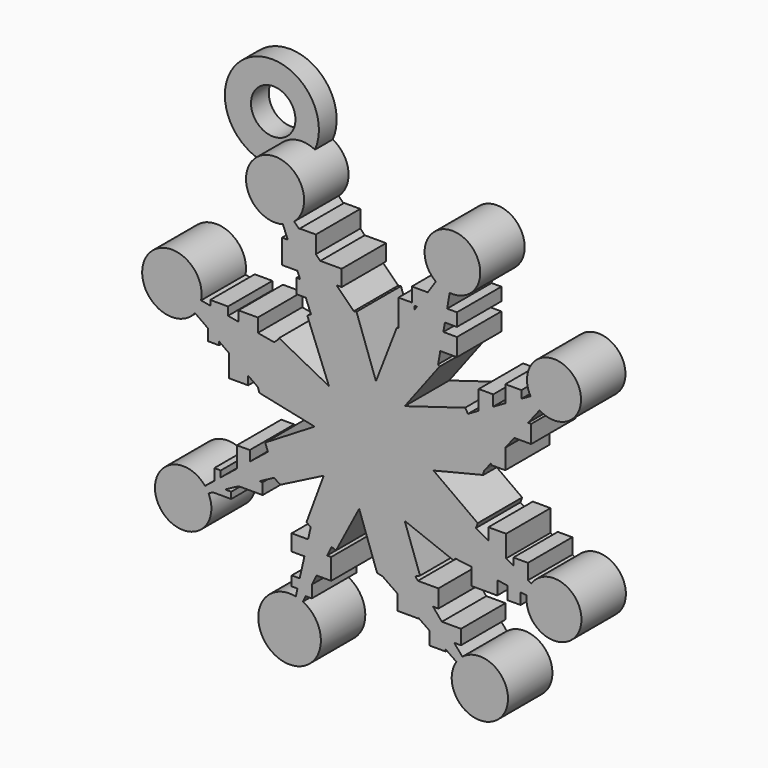
from build123d import *

# Parameters (mm, degrees)
F0_R      = 12.7857762136
F1_DEPTH  = 6.35
F3_DEPTH  = 6.35
F4_R      = 3.3993359565
F4_R_2    = 3.3235048552
F4_R_3    = 3.1824573901
F4_R_4    = 3.2248919367
F4_R_5    = 3.0903500786
F4_R_6    = 3.1394498191
F4_R_7    = 3.2196174713
F4_R_8    = 3.5795247409
F5_DEPTH  = 6.35
F7_DEPTH  = 75
F9_DEPTH  = 6.351
F10_W     = 2.0279027522
F10_H     = 1.2904834002
F10_W_2   = 2.2122580558
F10_H_2   = 2.5809677318
F10_W_3   = 1.8435483798
F10_H_3   = 2.0279027522
F10_W_4   = 2.7653225698
F10_H_4   = 1.8435493112
F10_W_5   = 2.5809649378
F10_H_5   = 1.4748387039
F10_W_6   = 2.0279064775
F10_H_6   = 2.0279036835
F10_W_7   = 1.6591902822
F10_H_7   = 2.3966128938
F10_W_8   = 1.6591958702
F10_H_8   = 3.502741456
F10_W_9   = 1.8435474485
F10_H_9   = 2.3966114968
F10_W_10  = 3.5027395934
F10_W_11  = 2.0278980955
F10_H_10  = 1.8435474485
F10_W_12  = 1.4748387039
F10_H_11  = 2.7653221041
F10_H_12  = 2.7653239667
F10_W_13  = 1.8435493112
F10_H_13  = 1.6591940075
F10_W_14  = 1.2904852629
F10_H_14  = 2.9496771749
F10_W_15  = 1.0139523074
F10_H_15  = 0.6452444941
F10_W_16  = 0.8295960724
F10_H_16  = 0.2765338868
F10_W_17  = 2.9496746138
F10_H_17  = 2.0279046148
F10_W_18  = 2.3966133595
F10_H_18  = 1.6591921449
F10_W_19  = 1.1061290279
F10_H_19  = 1.6591958702
F10_H_20  = 2.3966096342
F12_DEPTH = 6.35
F11_W     = 2.2122561932
F11_H     = 0.7374193519
F11_W_2   = 2.9496755451
F11_H_2   = 1.2904852629
F11_W_3   = 2.3966133595
F11_H_3   = 2.7653221041
F11_W_4   = 1.8435521051
F11_H_4   = 1.6591958702
F11_W_5   = 3.3183861524
F11_H_5   = 1.8435474485
F11_W_6   = 1.2904834002
F11_H_6   = 1.1061280966
F11_W_7   = 1.8250197172
F11_H_7   = 4.4321902096
F13_DEPTH = 6.35
F14_R     = 5.3746391735
F16_DEPTH = 2.54
F17_D     = 5.08
F18_SCALE = 0.8


# Not quite as in the source:
# - an extrude ends at something that could not be found from the text; its depth is read off the source's solid


with BuildPart() as f1:
    # F0 (on Front) → F1 (new body)
    with BuildSketch(Plane.XZ):
        Circle(F0_R)
    extrude(amount=F1_DEPTH)

    # F2 (on Front) → F3 (join)
    with BuildSketch(Plane.XZ):
        Polygon((-23.2665110379, 8.706712164), (-13.0349704996, 1.4206155902), (-11.1746909097, -4.1602244601), (-22.1813470125, -12.9965534434), (-11.1746909097, -7.1056671441), (-6.8340380676, -10.0511107594), (-9.4694346189, -21.6778609902), (-4.5086885802, -11.7563670501), (1.2271746527, -12.9965534434), (12.853924185, -21.0577659309), (4.9477354623, -11.7563670501), (9.5984349027, -8.5008768365), (21.5352289379, -10.0511107594), (10.9936436638, -4.1602244601), (12.853924185, 1.4206155902), (21.5352289379, 12.5822946429), (10.9936436638, 6.5363855101), (7.583131548, 10.4119684547), (9.5984349027, 22.0387186855), (3.2424782403, 12.5822946429), (-2.0283141639, 12.5822946429), (-11.484737508, 22.0387186855), (-6.8340380676, 10.4119684547), (-11.1746909097, 6.5363855101), align=None)
    extrude(amount=F3_DEPTH)

    # F4 (on Front) → F5 (join)
    with BuildSketch(Plane.XZ):
        with Locations((-22.85999991, 8.6646778509)):
            Circle(F4_R)
        with Locations((-11.061290279, 21.9382271171)):
            Circle(F4_R_2)
        with Locations((9.2177418992, 21.2008059025)):
            Circle(F4_R_3)
        with Locations((-21.5695165098, -12.5361289829)):
            Circle(F4_R_4)
        with Locations((20.8320971578, 12.1674193069)):
            Circle(F4_R_5)
        with Locations((20.8320971578, -9.9551612511)):
            Circle(F4_R_6)
        with Locations((12.3517736793, -20.6477418542)):
            Circle(F4_R_7)
        with Locations((-9.4020972028, -21.7538699508)):
            Circle(F4_R_8)
    extrude(amount=F5_DEPTH)

    # F6 (on Front) → F7 (cut, through all)
    with BuildSketch(Plane.XZ):
        Polygon((-7.5585483573, 10.1395165548), (-11.2456455827, 6.4524193294), (-5.5306456052, 3.6870969925), align=None)
    extrude(amount=-F7_DEPTH, mode=Mode.SUBTRACT)

    # F8 (on Front) → F9 (cut, through all)
    with BuildSketch(Plane.XZ):
        Polygon((-7.747462485, 11.3888066262), (-11.6853228265, 7.7033734991), (-4.8973932862, 4.1540157981), align=None)
        Polygon((3.10472399, 13.197503984), (-1.9377060235, 13.197503984), (0.4738910357, 6.401185412), align=None)
        Polygon((11.4356949925, 7.2781299241), (8.0375354737, 10.6214806437), (3.7624323741, 4.9595900422), align=None)
        Polygon((12.9703478888, -4.7250459902), (13.2992016152, 1.0847104713), (7.0509738289, -0.4499422212), align=None)
        Polygon((3.7624323741, -6.5885526128), (5.6807477959, -12.0146451518), (10.5650918246, -9.2218401007), align=None)
        Polygon((-1.4460915438, -7.060531742), (-4.2944937013, -12.5079266727), (0.8164772162, -13.4603694996), align=None)
        Polygon((-6.5416637808, -0.4499422212), (-13.7764541432, 1.0847104713), (-13.2831735536, -4.560619127), align=None)
        Polygon((-5.5002924055, -5.0539001822), (-11.200430803, -7.9587781802), (-8.076316677, -12.0146451518), align=None)
    extrude(amount=F9_DEPTH, mode=Mode.SUBTRACT)

    # F10 (on Front) → F12 (join)
    with BuildSketch(Plane.XZ):
        with Locations((-17.457537353, 7.7759893611)):
            Rectangle(F10_W, F10_H)
        with Locations((-14.1391512007, 7.1307471953)):
            Rectangle(F10_W_2, F10_H_2)
        with Locations((-7.3180221952, 17.9155059159)):
            Rectangle(F10_W_3, F10_H_3)
        with Locations((-4.8292321153, 15.5188925564)):
            Rectangle(F10_W_4, F10_H_4)
        with Locations((8.4443166852, 15.6110702083)):
            Rectangle(F10_W_5, F10_H_5)
        with Locations((17.2011721879, 6.8542151712)):
            Rectangle(F10_W_6, F10_H_6)
        with Locations((14.4358500838, 3.4436504357)):
            Rectangle(F10_W_7, F10_H_7)
        with Locations((13.0531890318, 7.6838117093)):
            Rectangle(F10_W_8, F10_H_8)
        with Locations((16.1872189492, 9.7117153928)):
            Rectangle(F10_W_9, F10_H_9)
        with Locations((7.9834293574, 12.8457471728)):
            Rectangle(F10_W_10, F10_H_3)
        with Locations((5.5868155323, 16.3484895602)):
            Rectangle(F10_W_11, F10_H_10)
        with Locations((-14.6922152489, -6.6036880016)):
            Rectangle(F10_W_12, F10_H_11)
        Polygon((-17.273183912, -9.8298983648), (-17.273183912, -8.355059661), (-18.0106014013, -8.355059661), (-18.0106014013, -10.5673158541), align=None)
        with Locations((-9.3459254131, 15.9797798842)):
            Rectangle(F10_W_9, F10_H_12)
        with Locations((-7.6867314056, 13.0301024765)):
            Rectangle(F10_W_13, F10_H_13)
        with Locations((-18.1027799845, 4.9184891395)):
            Rectangle(F10_W_14, F10_H_5)
        with Locations((-15.2452802286, 2.7062310837)):
            Rectangle(F10_W_2, F10_H_14)
        Polygon((15.3576238081, -7.4332859367), (15.3576238081, -4.1148979217), (13.3297191933, -4.1148979217), (13.3297191933, -6.7880414426), (14.3436715007, -6.7880414426), (14.3436715007, -7.4332859367), align=None)
        with Locations((13.836695347, -7.1106636897)):
            Rectangle(F10_W_15, F10_H_15)
        Polygon((13.3297191933, -7.4332859367), (13.3297191933, -6.7880414426), (11.3939959556, -6.7880414426), (11.3939959556, -10.6594953686), (14.3436715007, -10.6594953686), (14.3436715007, -7.4332859367), align=None)
        Polygon((17.846416682, -6.2349783257), (16.1872208118, -6.2349783257), (16.1872208118, -8.170703426), (17.0168168843, -8.170703426), (17.0168168843, -8.4472373128), (17.846416682, -8.4472373128), align=None)
        with Locations((16.6020188481, -8.3089703694)):
            Rectangle(F10_W_16, F10_H_16)
        Polygon((16.1872208118, -8.4472373128), (16.1872208118, -8.170703426), (15.5419781804, -8.170703426), (15.5419781804, -10.7516720891), (17.0168168843, -10.7516720891), (17.0168168843, -8.4472373128), align=None)
        with Locations((6.1398823746, -13.1482854486)):
            Rectangle(F10_W_17, F10_H_17)
        with Locations((8.9973807335, -16.1901395768)):
            Rectangle(F10_W_18, F10_H_18)
        with Locations((-7.4101993814, -17.0197356492)):
            Rectangle(F10_W_19, F10_H_19)
        with Locations((-5.8431830257, -14.162237756)):
            Rectangle(F10_W_18, F10_H_20)
    extrude(amount=F12_DEPTH)

    # F11 (on Front) → F13 (join)
    with BuildSketch(Plane.XZ):
        with Locations((-17.1810053289, -10.475140065)):
            Rectangle(F11_W, F11_H)
        with Locations((-13.954795897, -8.6315916851)):
            Rectangle(F11_W_2, F11_H_2)
        with Locations((4.1119782254, -14.5309465006)):
            Rectangle(F11_W_3, F11_H_3)
        with Locations((7.5225434266, -17.3884462565)):
            Rectangle(F11_W_4, F11_H_4)
        with Locations((-7.5023770332, -12.9639301449)):
            Rectangle(F11_W_5, F11_H_5)
        with Locations((-8.5163284093, -16.8353822082)):
            Rectangle(F11_W_6, F11_H_6)
        with Locations((3.9568627253, 13.4398583323)):
            Rectangle(F11_W_7, F11_H_7)
    extrude(amount=F13_DEPTH)

    # F14 (on Front) → F16 (join)
    with BuildSketch(Plane.XZ):
        with Locations((-14.4751127809, 27.0408820361)):
            Circle(F14_R)
    extrude(amount=F16_DEPTH)

    # F17 (through all)
    with Locations(Plane(origin=(0, 0, 0), x_dir=(1, 0, 0), z_dir=(0, 1, 0))):
        with Locations((-14.3200894818, -27.1959044039)):
            Hole(F17_D / 2)


with BuildPart() as f1_1:
    # F18: moved
    add(f1.part.scale(F18_SCALE))


solid = f1_1.part
